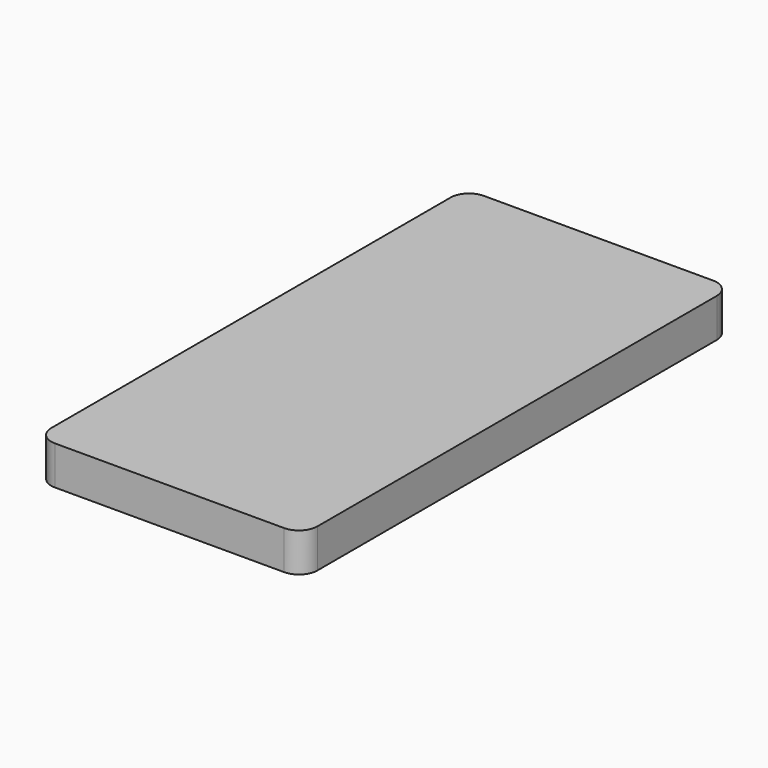
from build123d import *

# Parameters (mm, degrees)
F0_W     = 145
F0_H     = 10.5
F1_DEPTH = 36
F2_R     = 5
F3_T     = 5
F4_R     = 5


# Not quite as in the source:
# - a shell that OpenCascade refuses in one call is made with other operations: the cavity is built on its own and cut out


with BuildPart() as f1:
    # F0 (on Right) → F1 (new body, symmetric)
    with BuildSketch(Plane.YZ):
        Rectangle(F0_W, F0_H)
    extrude(amount=F1_DEPTH, both=True)

    # F2
    f2_edges = [f1.edges().sort_by_distance(p)[0] for p in [
        (36, -72.5, 0),
        (36, 72.5, 0),
        (-36, -72.5, 0),
        (-36, 72.5, 0),
    ]]
    fillet(f2_edges, radius=F2_R)

    # F3: shell of thickness 5, made by hand


with BuildPart() as f3_core1:
    # F3_t2: copy of F1
    add(f1.part)

    # the walls: a layer under each face that stays
    f3_faces = [f3_core1.faces().sort_by_distance(p)[0] for p in [
        (-36, 0, 0),
        (0, -72.5, 0),
        (0, 72.5, 0),
        (36, 0, 0),
        (0, 0, 5.25),
    ]]
    thicken(f3_faces, amount=-F3_T, mode=Mode.SUBTRACT)


with BuildPart() as f1_1:
    add(f1.part)

    # what is left inside the walls is the cavity
    f3_cavity = [f3_core1.part.solids().sort_by_distance(p)[0] for p in [
        (-10.333333, 0, -5.2),
    ]]
    add(f3_cavity, mode=Mode.SUBTRACT)

    # F4
    f4_edges = [f1_1.edges().sort_by_distance(p)[0] for p in [
        (-31, -67.5, -2.5),
        (31, -67.5, -2.5),
        (-31, 67.5, -2.5),
        (31, 67.5, -2.5),
    ]]
    fillet(f4_edges, radius=F4_R)


solid = f1_1.part
